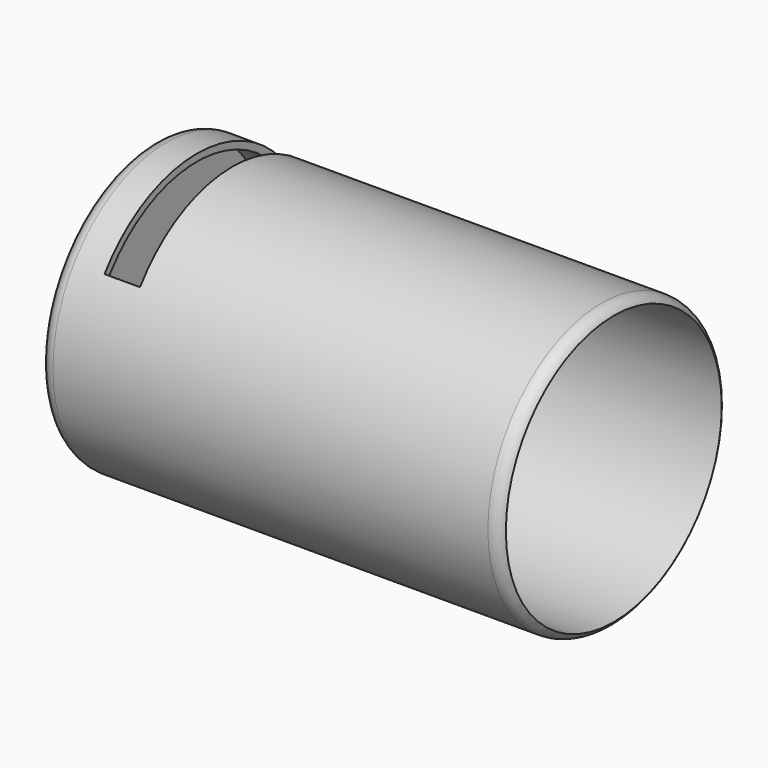
from build123d import *

# Parameters (mm, degrees)
F0_R     = 50.8
F1_DEPTH = 82.55
F2_T     = -2.54
F5_DEPTH = 152.4


# Not quite as in the source:
# - a fillet or chamfer that OpenCascade refuses, or shapes differently, is made with other operations: its cross-section is extruded or revolved along the edge and cut away or added


with BuildPart() as f1:
    # F0 (on Right) → F1 (new body, symmetric)
    with BuildSketch(Plane.YZ):
        Circle(F0_R)
    extrude(amount=F1_DEPTH, both=True)

    # F2
    f2_openings = [f1.faces().sort_by_distance(p)[0] for p in [
        (82.55, 0, 0),
    ]]
    offset(amount=F2_T, openings=f2_openings)

    # F3: fillet of radius 5.08 on 3 edges, made by hand

    # F3_s1 → F3_t2 (revolve, cut)
    with BuildSketch(Plane.XY):
        with BuildLine():
            ThreePointArc((-77.47, 50.8), (-81.0621024484, 49.3121024484), (-82.55, 45.72))
            Line((-82.55, 45.72), (-82.55, 50.8))
            Line((-82.55, 50.8), (-77.47, 50.8))
        make_face()
    revolve(axis=Axis((-82.55, 0, 0), (1, 0, 0)), mode=Mode.SUBTRACT)

    # F3_s3 → F3_t4 (revolve, cut)
    with BuildSketch(Plane.XY):
        with BuildLine():
            ThreePointArc((78.1505909488, 50.8), (80.6905909488, 50.1194090512), (82.55, 48.26))
            Line((82.55, 48.26), (82.55, 50.8))
            Line((82.55, 50.8), (78.1505909488, 50.8))
        make_face()
    revolve(axis=Axis((82.55, 0, 0), (1, 0, 0)), mode=Mode.SUBTRACT)

    # F4 (on Top) → F5 (cut)
    with BuildSketch(Plane.XY):
        Polygon((-53.9159391403, 0), (-53.9159391403, 41.275), (-66.6159391403, 41.275), (-66.6159391403, 0), (-66.6159391403, -41.275), (-53.9159391403, -41.275), align=None)
    extrude(amount=F5_DEPTH, mode=Mode.SUBTRACT)


solid = f1.part
